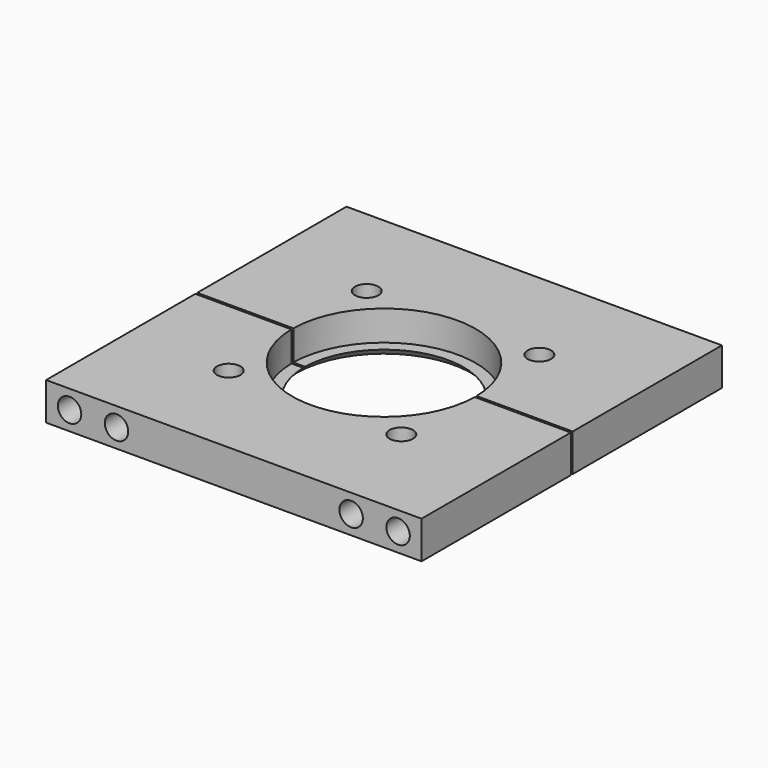
from build123d import *

# Parameters (mm, degrees)
F0_R          = 3.96875
F1_DEPTH      = 6.35
F2_DEPTH      = 3.81
F2_DEPTH_BACK = 6.35
F3_SIZE       = 2.53999
F3_2_SIZE     = 2.53999
F4_R          = 3.96875
F5_DEPTH      = 63.5


# Not quite as in the source:
# - a fillet or chamfer is up to 0.001 mm smaller than in the source, because OpenCascade refuses the exact size


with BuildPart() as f1:
    # F0 (on Top) → F1 (new body, symmetric)
    with BuildSketch(Plane.XY):
        with BuildLine():
            Line((26.9970829949, 0.396875), (30.9974594158, 0.396875))
            ThreePointArc((30.9974594158, 0.396875), (0, 31), (-30.9974594158, 0.396875))
            Line((-30.9974594158, 0.396875), (-26.9970829949, 0.396875))
            ThreePointArc((-26.9970829949, 0.396875), (0, 27), (26.9970829949, 0.396875))
        make_face()
        with BuildLine():
            ThreePointArc((-30.9974594158, 0.396875), (0, 31), (30.9974594158, 0.396875))
            Line((30.9974594158, 0.396875), (63.5, 0.396875))
            Line((63.5, 0.396875), (63.5, 63.5))
            Line((63.5, 63.5), (-63.5, 63.5))
            Line((-63.5, 63.5), (-63.5, 0.396875))
            Line((-63.5, 0.396875), (-30.9974594158, 0.396875))
        make_face()
        with Locations((-29.1858323935, 29.1858323935)):
            Circle(F0_R, mode=Mode.SUBTRACT)
        with Locations((29.1858323935, 29.1858323935)):
            Circle(F0_R, mode=Mode.SUBTRACT)
    extrude(amount=F1_DEPTH, both=True)


with BuildPart() as f1b:
    # F0 (on Top) → F1, piece 2 (new body, symmetric)
    with BuildSketch(Plane.XY):
        with BuildLine():
            Line((63.5, -0.396875), (30.9974594158, -0.396875))
            ThreePointArc((30.9974594158, -0.396875), (0, -31), (-30.9974594158, -0.396875))
            Line((-30.9974594158, -0.396875), (-63.5, -0.396875))
            Line((-63.5, -0.396875), (-63.5, -63.5))
            Line((-63.5, -63.5), (63.5, -63.5))
            Line((63.5, -63.5), (63.5, -0.396875))
        make_face()
        with Locations((-29.1858323935, -29.1858323935)):
            Circle(F0_R, mode=Mode.SUBTRACT)
        with Locations((29.1858323935, -29.1858323935)):
            Circle(F0_R, mode=Mode.SUBTRACT)
        with BuildLine():
            ThreePointArc((-30.9974594158, -0.396875), (0, -31), (30.9974594158, -0.396875))
            Line((30.9974594158, -0.396875), (26.9970829949, -0.396875))
            ThreePointArc((26.9970829949, -0.396875), (0, -27), (-26.9970829949, -0.396875))
            Line((-26.9970829949, -0.396875), (-30.9974594158, -0.396875))
        make_face()
    extrude(amount=F1_DEPTH, both=True)


with BuildPart() as f2_tool:
    # F0 (on Top) → F2 (new body, two sides)
    with BuildSketch(Plane.XY) as f2_sk:
        with BuildLine():
            ThreePointArc((-30.9974594158, -0.396875), (0, -31), (30.9974594158, -0.396875))
            Line((30.9974594158, -0.396875), (26.9970829949, -0.396875))
            ThreePointArc((26.9970829949, -0.396875), (0, -27), (-26.9970829949, -0.396875))
            Line((-26.9970829949, -0.396875), (-30.9974594158, -0.396875))
        make_face()
        with BuildLine():
            Line((26.9970829949, 0.396875), (30.9974594158, 0.396875))
            ThreePointArc((30.9974594158, 0.396875), (0, 31), (-30.9974594158, 0.396875))
            Line((-30.9974594158, 0.396875), (-26.9970829949, 0.396875))
            ThreePointArc((-26.9970829949, 0.396875), (0, 27), (26.9970829949, 0.396875))
        make_face()
    extrude(amount=-F2_DEPTH)
    extrude(f2_sk.sketch, amount=F2_DEPTH_BACK)


with BuildPart() as f1_1:
    add(f1.part)

    # F2: cut by f2_tool
    add(f2_tool.part, mode=Mode.SUBTRACT)

    # F3 (size 2.54 in the source; OpenCascade refuses exactly that, so slightly less here)
    f3_edges = [f1_1.edges().sort_by_distance(p)[0] for p in [
        (0, 27, -6.35),
    ]]
    chamfer(f3_edges, length=F3_SIZE)


with BuildPart() as f1b_1:
    add(f1b.part)

    # F2: cut by f2_tool
    add(f2_tool.part, mode=Mode.SUBTRACT)

    # F3#2 (size 2.54 in the source; OpenCascade refuses exactly that, so slightly less here)
    f3_2_edges = [f1b_1.edges().sort_by_distance(p)[0] for p in [
        (0, -27, -6.35),
    ]]
    chamfer(f3_2_edges, length=F3_2_SIZE)


with BuildPart() as f5_tool:
    # F4 (on Front) → F5 (new body, symmetric)
    with BuildSketch(Plane.XZ):
        with BuildLine():
            ThreePointArc((43.65625, 0), (39.6875, 3.96875), (35.71875, 0))
            ThreePointArc((35.71875, 0), (39.6875, -3.96875), (43.65625, 0))
        make_face()
        with Locations((55.5625, 0)):
            Circle(F4_R)
        with Locations((-39.6875, 0)):
            Circle(F4_R)
        with Locations((-55.5625, 0)):
            Circle(F4_R)
    extrude(amount=F5_DEPTH, both=True)


with BuildPart() as f1_2:
    add(f1_1.part)

    # F5: cut by f5_tool
    add(f5_tool.part, mode=Mode.SUBTRACT)


with BuildPart() as f1b_2:
    add(f1b_1.part)

    # F5: cut by f5_tool
    add(f5_tool.part, mode=Mode.SUBTRACT)


solid = Compound([f1_2.part, f1b_2.part])
